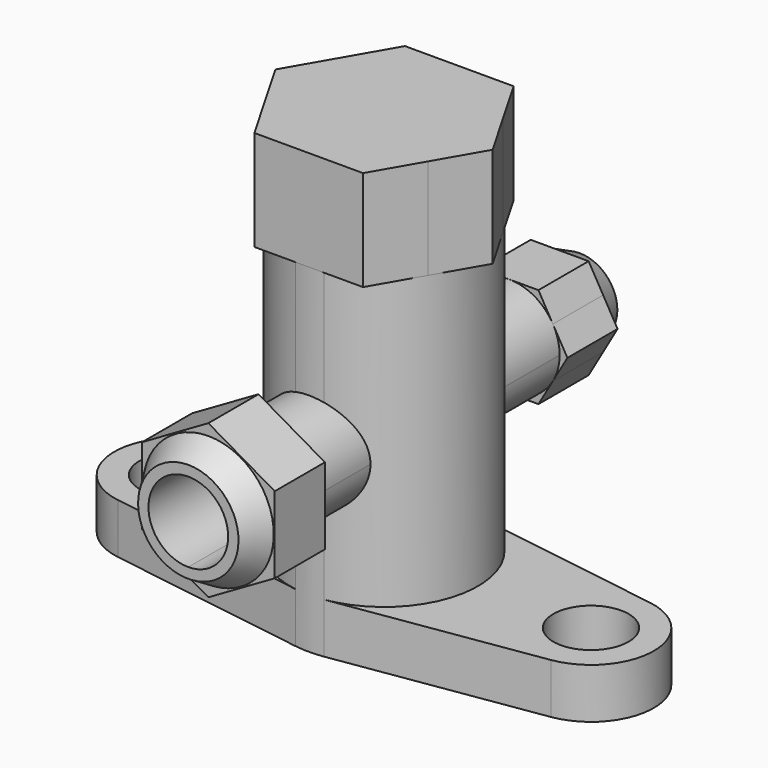
from build123d import *
from build123d import SkipClean  # not in build123d's __all__

# Parameters (mm, degrees)
F0_R      = 3
F1_DEPTH  = 4
F0_R_2    = 3.175
F2_DEPTH  = 27
F3_R      = 3.175
F4_DEPTH  = 8
F6_R      = 5.7217955199
F6_R_2    = 3.175
F7_DEPTH  = 8
F9_DEPTH  = 17.5
F10_DEPTH = 18
F11_R     = 4
F11_R_2   = 3.175
F12_DEPTH = 5
F13_R     = 3.175
F14_DEPTH = 5
F17_DEPTH = 19.5


with BuildPart() as f1:
    # F0 (on Top) → F1 (new body)
    with BuildSketch(Plane.XY):
        with BuildLine():
            ThreePointArc((-1.1363636364, -7.4134120138), (-7.5, 0), (-1.1363636364, 7.4134120138))
            Line((-1.1363636364, 7.4134120138), (-17.2575757576, 4.9422746758))
            ThreePointArc((-17.2575757576, 4.9422746758), (-21.5, 0), (-17.2575757576, -4.9422746758))
            Line((-17.2575757576, -4.9422746758), (-1.1363636364, -7.4134120138))
        make_face()
        with Locations((-16.5, 0)):
            Circle(F0_R, mode=Mode.SUBTRACT)
    extrude(amount=F1_DEPTH)



with BuildPart() as f1b:
    # F0 (on Top) → F1, piece 2 (new body)
    with BuildSketch(Plane.XY):
        with BuildLine():
            ThreePointArc((1.1363636364, 7.4134120138), (5.6909018298, 4.8850421046), (7.5, 0))
            ThreePointArc((7.5, 0), (5.6909018298, -4.8850421046), (1.1363636364, -7.4134120138))
            Line((1.1363636364, -7.4134120138), (17.2575757576, -4.9422746758))
            ThreePointArc((17.2575757576, -4.9422746758), (21.5, 0), (17.2575757576, 4.9422746758))
            Line((17.2575757576, 4.9422746758), (1.1363636364, 7.4134120138))
        make_face()
        with Locations((16.5, 0)):
            Circle(F0_R, mode=Mode.SUBTRACT)
    extrude(amount=F1_DEPTH)


with BuildPart() as f1_1:
    add(f1.part, clean=False)

    add(f1b.part)  # F2 merges F1b
    # F0 (on Top) → F2 (join)
    with BuildSketch(Plane.XY):
        with BuildLine():
            ThreePointArc((1.1363636364, -7.4134120138), (5.6909018298, -4.8850421046), (7.5, 0))
            ThreePointArc((7.5, 0), (5.6909018298, 4.8850421046), (1.1363636364, 7.4134120138))
            ThreePointArc((1.1363636364, 7.4134120138), (0, 7.5), (-1.1363636364, 7.4134120138))
            ThreePointArc((-1.1363636364, 7.4134120138), (-7.5, 0), (-1.1363636364, -7.4134120138))
            ThreePointArc((-1.1363636364, -7.4134120138), (0, -7.5), (1.1363636364, -7.4134120138))
        make_face()
        Circle(F0_R_2, mode=Mode.SUBTRACT)
    extrude(amount=F2_DEPTH)

    # F3 (on face) → F4 (join)
    with BuildSketch(Plane.XY.offset(27)):
        with BuildLine():
            ThreePointArc((-6.4951910722, -3.749999058), (-3.750000471, -6.4951902565), (0, -7.5))
            ThreePointArc((0, -7.5), (3.7500004715, -6.4951902561), (6.4951910729, -3.7499990569))
            ThreePointArc((6.4951910729, -3.7499990569), (7.2444438381, -1.9411423123), (7.5, 0))
            ThreePointArc((7.5, 0), (7.2444437844, 1.9411425128), (6.4951908653, 3.7499994165))
            ThreePointArc((6.4951908653, 3.7499994165), (3.7500002918, 6.4951903599), (0, 7.5))
            ThreePointArc((0, 7.5), (-3.750000255, 6.4951903812), (-6.4951908228, 3.7499994901))
            ThreePointArc((-6.4951908228, 3.7499994901), (-7.5, 2.494e-07), (-6.4951910722, -3.749999058))
        make_face()
        Circle(F3_R, mode=Mode.SUBTRACT)
        with BuildLine():
            Line((-4.3301270189, -7.5), (0, -7.5))
            ThreePointArc((0, -7.5), (-3.750000471, -6.4951902565), (-6.4951910722, -3.749999058))
            Line((-6.4951910722, -3.749999058), (-4.3301270189, -7.5))
        make_face()
        with BuildLine():
            Line((-8.6602540378, 0), (-6.4951910722, -3.749999058))
            ThreePointArc((-6.4951910722, -3.749999058), (-7.5, 2.494e-07), (-6.4951908228, 3.7499994901))
            Line((-6.4951908228, 3.7499994901), (-8.6602540378, 0))
        make_face()
        with BuildLine():
            Line((0, -7.5), (4.3301270189, -7.5))
            Line((4.3301270189, -7.5), (6.4951910729, -3.7499990569))
            ThreePointArc((6.4951910729, -3.7499990569), (3.7500004715, -6.4951902561), (0, -7.5))
        make_face()
        with BuildLine():
            ThreePointArc((7.5, 0), (7.2444438381, -1.9411423123), (6.4951910729, -3.7499990569))
            Line((6.4951910729, -3.7499990569), (8.6602540378, 0))
            Line((8.6602540378, 0), (6.4951908653, 3.7499994165))
            ThreePointArc((6.4951908653, 3.7499994165), (7.2444437844, 1.9411425128), (7.5, 0))
        make_face()
        with BuildLine():
            ThreePointArc((0, 7.5), (3.7500002918, 6.4951903599), (6.4951908653, 3.7499994165))
            Line((6.4951908653, 3.7499994165), (4.3301270189, 7.5))
            Line((4.3301270189, 7.5), (0, 7.5))
        make_face()
        with BuildLine():
            Line((-4.3301270189, 7.5), (-6.4951908228, 3.7499994901))
            ThreePointArc((-6.4951908228, 3.7499994901), (-3.750000255, 6.4951903812), (0, 7.5))
            Line((0, 7.5), (-4.3301270189, 7.5))
        make_face()
    extrude(amount=F4_DEPTH)

    # F6 (on face) → F7 (join)
    with BuildSketch(Plane.XY.offset(35)):
        Circle(F6_R)
        Circle(F6_R_2, mode=Mode.SUBTRACT)
        Circle(F6_R_2)
    extrude(amount=-F7_DEPTH)

    # F8 (on Front) → F9 (join, symmetric)
    with BuildSketch(Plane.XZ):
        with BuildLine():
            ThreePointArc((4, 14), (-2.8284271247, 16.8284271247), (0, 10))
            ThreePointArc((0, 10), (2.8284271247, 11.1715728753), (4, 14))
        make_face()
        with BuildLine():
            ThreePointArc((3.175, 14), (2.2450640303, 11.7549359697), (0, 10.825))
            ThreePointArc((0, 10.825), (-2.2450640303, 16.2450640303), (3.175, 14))
        make_face(mode=Mode.SUBTRACT)
    extrude(amount=F9_DEPTH, both=True)

    # F0 (on Top) → F10 (cut)
    with BuildSketch(Plane.XY):
        Circle(F0_R_2)
    extrude(amount=F10_DEPTH, mode=Mode.SUBTRACT)

    # F11 (on face) → F12 (join)
    with BuildSketch(Plane.XZ.offset(17.5)):
        Polygon((5.2903494798, 10.9456153038), (5.2903494798, 17.0543846962), (0, 20.1087693925), (-5.2903494798, 17.0543846962), (-5.2903494798, 10.9456153038), (0, 7.8912306075), align=None)
        with Locations((0, 14)):
            Circle(F11_R, mode=Mode.SUBTRACT)
        with Locations((0, 14)):
            Circle(F11_R_2)
    extrude(amount=-F12_DEPTH)

    # F13 (on face) → F14 (join)
    with BuildSketch(Plane(origin=(0, 17.5, 0), x_dir=(-1, 0, 0), z_dir=(0, 1, 0))):
        with BuildLine():
            ThreePointArc((-3.4641015674, 11.9999999173), (-1.9999999587, 10.535898361), (0, 10))
            ThreePointArc((0, 10), (1.9999999969, 10.5358983831), (3.4641016116, 11.9999999938))
            ThreePointArc((3.4641016116, 11.9999999938), (3.8637033042, 12.9647238161), (4, 14))
            ThreePointArc((4, 14), (3.8637033227, 15.0352761149), (3.464101683, 15.9999998825))
            ThreePointArc((3.464101683, 15.9999998825), (2.0000000588, 17.4641015812), (0, 18))
            ThreePointArc((0, 18), (-1.9999999587, 17.464101639), (-3.4641015674, 16.0000000827))
            ThreePointArc((-3.4641015674, 16.0000000827), (-4, 14), (-3.4641015674, 11.9999999173))
        make_face()
        with Locations((0, 14)):
            Circle(F13_R, mode=Mode.SUBTRACT)
        with Locations((0, 14)):
            Circle(F13_R)
        with BuildLine():
            ThreePointArc((4, 14), (3.8637033042, 12.9647238161), (3.4641016116, 11.9999999938))
            Line((3.4641016116, 11.9999999938), (4.6188021535, 14))
            Line((4.6188021535, 14), (3.464101683, 15.9999998825))
            ThreePointArc((3.464101683, 15.9999998825), (3.8637033227, 15.0352761149), (4, 14))
        make_face()
        with BuildLine():
            ThreePointArc((0, 18), (2.0000000588, 17.4641015812), (3.464101683, 15.9999998825))
            Line((3.464101683, 15.9999998825), (2.3094010768, 18))
            Line((2.3094010768, 18), (0, 18))
        make_face()
        with BuildLine():
            Line((-2.3094010768, 18), (-3.4641015674, 16.0000000827))
            ThreePointArc((-3.4641015674, 16.0000000827), (-1.9999999587, 17.464101639), (0, 18))
            Line((0, 18), (-2.3094010768, 18))
        make_face()
        with BuildLine():
            Line((-4.6188021535, 14), (-3.4641015674, 11.9999999173))
            ThreePointArc((-3.4641015674, 11.9999999173), (-4, 14), (-3.4641015674, 16.0000000827))
            Line((-3.4641015674, 16.0000000827), (-4.6188021535, 14))
        make_face()
        with BuildLine():
            Line((-2.3094010768, 10), (0, 10))
            ThreePointArc((0, 10), (-1.9999999587, 10.535898361), (-3.4641015674, 11.9999999173))
            Line((-3.4641015674, 11.9999999173), (-2.3094010768, 10))
        make_face()
        with BuildLine():
            Line((0, 10), (2.3094010768, 10))
            Line((2.3094010768, 10), (3.4641016116, 11.9999999938))
            ThreePointArc((3.4641016116, 11.9999999938), (1.9999999969, 10.5358983831), (0, 10))
        make_face()
    extrude(amount=-F14_DEPTH)

    # F15 (on Right) → F16 (revolve)
    with BuildSketch(Plane.YZ):
        Polygon((17.5, 18), (17.5, 14), (19.5, 14), (19.5, 17), align=None)
        Polygon((-19.5, 14), (-17.5, 14), (-17.5, 19.2129127681), (-19.5, 18), align=None)
    revolve(axis=Axis((0, -18.5, 14), (0, -1, 0)))

    # F8 (on Front) → F17 (cut, through all)
    with BuildSketch(Plane.XZ):
        with BuildLine():
            ThreePointArc((3.175, 14), (-2.2450640303, 16.2450640303), (0, 10.825))
            ThreePointArc((0, 10.825), (2.2450640303, 11.7549359697), (3.175, 14))
        make_face()
    with SkipClean():  # cleaning this boolean's faces spoils the solid; the shape is the same uncleaned
        extrude(amount=F17_DEPTH, mode=Mode.SUBTRACT)


solid = f1_1.part
